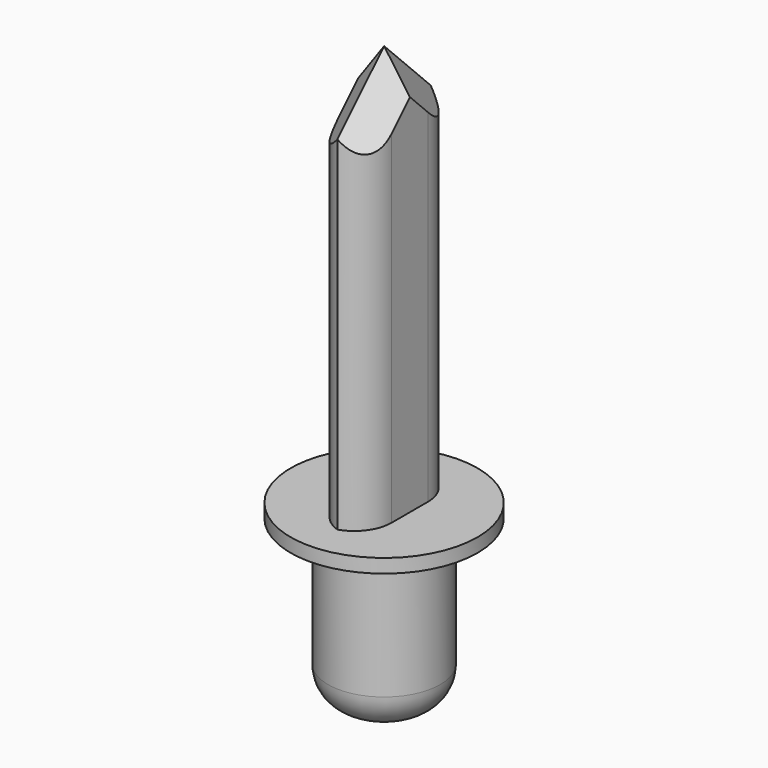
from build123d import *

# Parameters (mm, degrees)
F0_R         = 63.5
F1_DEPTH     = 9.398
F2_R         = 38.1
F3_DEPTH     = 111.506
F4_W         = 35.051997751
F4_H         = 81.7880034447
F5_DEPTH     = 304.8
F6_R         = 24.5284097937
F7_T1_DEPTH  = 296.3349893283
F8_T1_DEPTH  = 227.6667963807
F8_T3_DEPTH  = 227.6667963807
F9_T1_DEPTH  = 194.6467963807
F9_T3_DEPTH  = 194.6467963807
F10_T1_DEPTH = 270.8026681705


# Not quite as in the source:
# - a fillet or chamfer that OpenCascade refuses, or shapes differently, is made with other operations: its cross-section is extruded or revolved along the edge and cut away or added


with BuildPart() as f1:
    # F0 (on Top) → F1 (new body)
    with BuildSketch(Plane.XY):
        Circle(F0_R)
    extrude(amount=F1_DEPTH)

    # F2 (on face) → F3 (join)
    with BuildSketch(Plane(origin=(0, 0, 0), x_dir=(1, 0, 0), z_dir=(0, 0, -1))):
        Circle(F2_R)
    extrude(amount=F3_DEPTH)

    # F4 (on face) → F5 (join)
    with BuildSketch(Plane.XY.offset(9.398)):
        Rectangle(F4_W, F4_H)
    extrude(amount=F5_DEPTH)

    # F6
    f6_edges = [f1.edges().sort_by_distance(p)[0] for p in [
        (-38.1, 0, -111.506),
    ]]
    fillet(f6_edges, radius=F6_R)

    # F7: chamfer of 50.8 on 2 edges, made by hand

    # F7_s2 → F7_t1 (cut)
    with BuildSketch(Plane.YZ.offset(-148.1674946642)):
        Polygon((40.8940017223, 263.398), (-9.9059982777, 314.198), (40.8940017223, 314.198), align=None)
        Polygon((-40.8940017223, 263.398), (9.9059982777, 314.198), (-40.8940017223, 314.198), align=None)
    extrude(amount=F7_T1_DEPTH, mode=Mode.SUBTRACT)

    # F8: chamfer of 33.02 on 2 edges, made by hand

    # F8_s2 → F8_t1 (cut)
    with BuildSketch(Plane(origin=(0, -51.2066322141, 51.2066322141), x_dir=(1, 0, 0), z_dir=(0, -0.7071067812, 0.7071067812))):
        Polygon((17.5259988755, 182.1469378787), (-15.4940011245, 215.1669378787), (17.5259988755, 215.1669378787), align=None)
    extrude(amount=F8_T1_DEPTH, mode=Mode.SUBTRACT)

    # F8_s4 → F8_t3 (cut)
    with BuildSketch(Plane(origin=(0, -212.1913677859, 212.1913677859), x_dir=(1, 0, 0), z_dir=(0, 0.7071067812, -0.7071067812))):
        Polygon((-17.5259988755, -182.1469378787), (15.4940011245, -215.1669378787), (-17.5259988755, -215.1669378787), align=None)
    extrude(amount=F8_T3_DEPTH, mode=Mode.SUBTRACT)

    # F9: chamfer of 33.02 on 2 edges, made by hand

    # F9_s2 → F9_t1 (cut)
    with BuildSketch(Plane(origin=(0, 188.8427018711, 188.8427018711), x_dir=(1, 0, 0), z_dir=(0, -0.7071067812, -0.7071067812))):
        Polygon((-17.5259988755, 182.1469378787), (15.4940011245, 215.1669378787), (-17.5259988755, 215.1669378787), align=None)
    extrude(amount=F9_T1_DEPTH, mode=Mode.SUBTRACT)

    # F9_s4 → F9_t3 (cut)
    with BuildSketch(Plane(origin=(0, 51.2066322141, 51.2066322141), x_dir=(1, 0, 0), z_dir=(0, 0.7071067812, 0.7071067812))):
        Polygon((17.5259988755, -182.1469378787), (-15.4940011245, -215.1669378787), (17.5259988755, -215.1669378787), align=None)
    extrude(amount=F9_T3_DEPTH, mode=Mode.SUBTRACT)

    # F10: fillet of radius 25.4 on 4 edges, made by hand

    # F10_s2 → F10_t1 (cut)
    with BuildSketch(Plane.XY.offset(9.398)):
        with BuildLine():
            ThreePointArc((7.8740011245, 40.8940017223), (-10.0865111176, 33.4545139645), (-17.5259988755, 15.4940017223))
            Line((-17.5259988755, 15.4940017223), (-17.5259988755, 40.8940017223))
            Line((-17.5259988755, 40.8940017223), (7.8740011245, 40.8940017223))
        make_face()
        with BuildLine():
            ThreePointArc((17.5259988755, 15.4940017223), (10.0865111176, 33.4545139645), (-7.8740011245, 40.8940017223))
            Line((-7.8740011245, 40.8940017223), (17.5259988755, 40.8940017223))
            Line((17.5259988755, 40.8940017223), (17.5259988755, 15.4940017223))
        make_face()
        with BuildLine():
            ThreePointArc((-17.5259988755, -15.4940017223), (-10.0865111176, -33.4545139645), (7.8740011245, -40.8940017223))
            Line((7.8740011245, -40.8940017223), (-17.5259988755, -40.8940017223))
            Line((-17.5259988755, -40.8940017223), (-17.5259988755, -15.4940017223))
        make_face()
        with BuildLine():
            ThreePointArc((17.5259988755, -15.4940017223), (10.0865111176, -33.4545139645), (-7.8740011245, -40.8940017223))
            Line((-7.8740011245, -40.8940017223), (17.5259988755, -40.8940017223))
            Line((17.5259988755, -40.8940017223), (17.5259988755, -15.4940017223))
        make_face()
    extrude(amount=F10_T1_DEPTH, mode=Mode.SUBTRACT)


solid = f1.part
